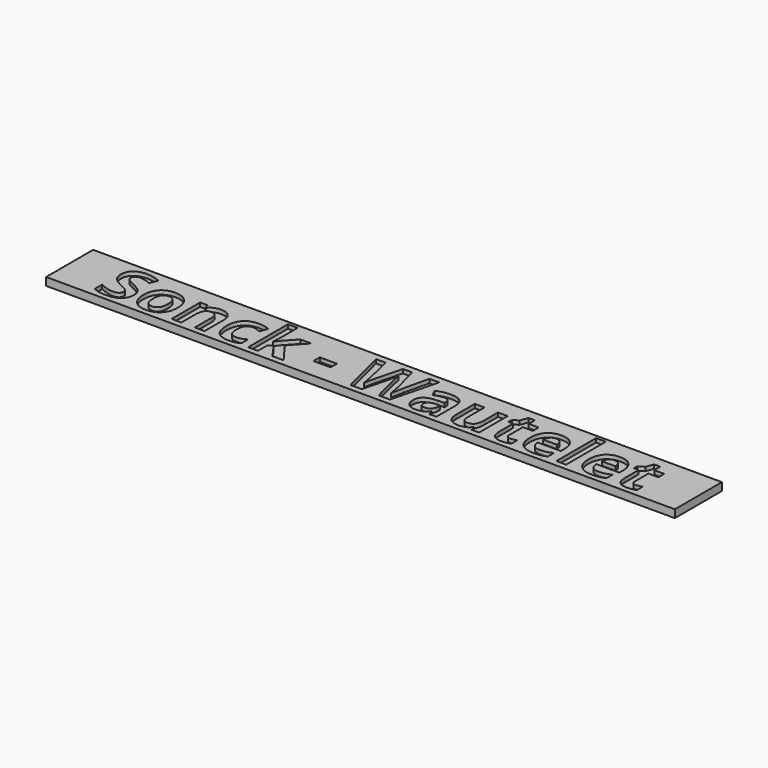
from build123d import *

# Parameters (mm, degrees)
F0_W         = 160.31
F0_H         = 15
F1_DEPTH     = 2
F3_TEXT_SIZE = 16.6666666667
F4_DEPTH     = 1


# Not quite as in the source:
# - Text() gives the source's letters only with a copy of the font that has no kerning and outlines rounded to 1/6400 em; it was checked with that copy


with BuildPart() as f1:
    # F0 (on Top) → F1 (new body)
    with BuildSketch(Plane.XY):
        with Locations((4.8425748038, -0.0022680685)):
            Rectangle(F0_W, F0_H)
    extrude(amount=F1_DEPTH)

    # F3 (on offset) → F4 (cut)
    with BuildSketch(Plane.XY.offset(2)):
        with Locations((-65.3124251962, -6.0018114352)):
            Text('Sonck - Wautelet', F3_TEXT_SIZE, font='Open Sans', font_style=FontStyle.BOLD, text_align=(TextAlign.LEFT, TextAlign.BOTTOM))
    extrude(amount=-F4_DEPTH, mode=Mode.SUBTRACT)


solid = f1.part
